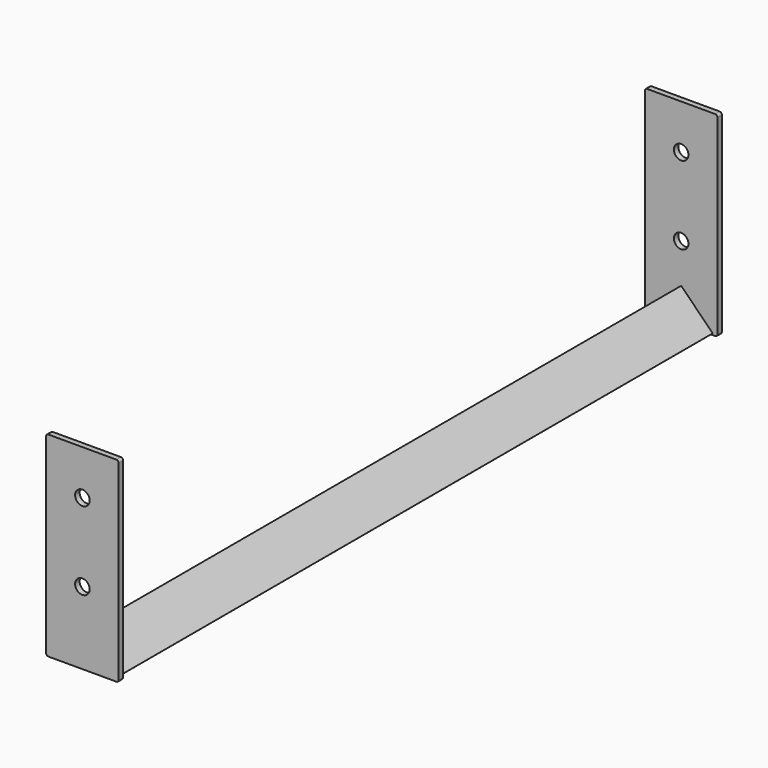
from build123d import *

# Parameters (mm, degrees)
F1_DEPTH      = 332.5
F1_DEPTH_BACK = 332.5
F2_R          = 4.99999
F3_W          = 65
F3_H          = 175
F4_DEPTH      = 5
F5_R          = 2
F7_D          = 13


# Not quite as in the source:
# - a fillet or chamfer is up to 0.001 mm smaller than in the source, because OpenCascade refuses the exact size
# - a pattern or mirror of a feature is missing from the dataset's text; its kind, count and spacing are read off the source's solid
# - a feature names something its author has since deleted; it is built from what else it names


with BuildPart() as f1:
    # F0 (on Front) → F1 (new body, two sides)
    with BuildSketch(Plane.XZ) as f1_sk:
        Polygon((0, 28.2842712475), (-28.2842712475, 0), (-24.7487373415, -3.5355339059), (0, 21.2132034356), (24.7487373415, -3.5355339059), (28.2842712475, 0), align=None)
    extrude(amount=F1_DEPTH)
    extrude(f1_sk.sketch, amount=-F1_DEPTH_BACK)

    # F2 (radius 5 in the source; OpenCascade refuses exactly that, so slightly less here)
    f2_edges = [f1.edges().sort_by_distance(p)[0] for p in [
        (24.748737, 0, -3.535534),
        (0, 0, 21.213203),
        (-24.748737, 0, -3.535534),
    ]]
    fillet(f2_edges, radius=F2_R)

    # F3 (on face) → F4 (join)
    with BuildSketch(Plane.XZ.offset(332.5)):
        with Locations((0, 86.0355339059)):
            Rectangle(F3_W, F3_H)
    f4 = extrude(amount=F4_DEPTH)

    # F4_copies: F4 across plane
    add(f4.mirror(Plane.ZX))

    # F5
    f5_edges = [f1.edges().sort_by_distance(p)[0] for p in [
        (32.5, -335, 173.535534),
        (32.5, -335, -1.464466),
        (-32.5, -335, 173.535534),
        (-32.5, -335, -1.464466),
        (-32.5, 335, -1.464466),
        (32.5, 335, -1.464466),
        (-32.5, 335, 173.535534),
        (32.5, 335, 173.535534),
    ]]
    fillet(f5_edges, radius=F5_R)

    # F7 (through all)
    with Locations(Plane.XZ.offset(337.5)):
        with Locations((0, 63.5355339059), (0, 133.5355339059)):
            Hole(F7_D / 2)


solid = f1.part
